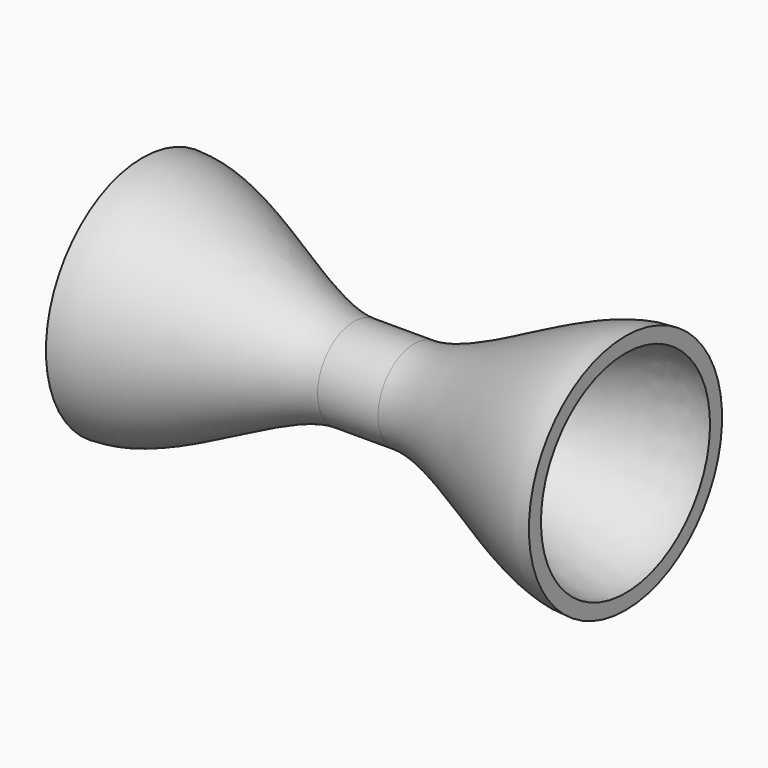
from build123d import *


# Not quite as in the source:
# - the dataset's text gives a spline's control points without its knots; the knots are read off the source's solid


with BuildPart() as f1:
    # F0 (on Front) → F1 (revolve)
    with BuildSketch(Plane.XZ):
        with BuildLine():
            Line((-66.7312243659, 73.4475515783), (-66.7312243659, 70.2725515783))
            add(Edge.make_bspline(
                [(-22.2812243659, 54.3975515783), (-34.9812243659, 54.3975515783), (-54.0312243659, 70.2725515783), (-66.7312243659, 70.2725515783)],
                knots=[0, 0, 0, 0, 47.1997682727, 47.1997682727, 47.1997682727, 47.1997682727], degree=3))
            Line((-22.2812243659, 54.3975515783), (-15.9312243659, 54.3975515783))
            Line((-15.9312243659, 54.3975515783), (-9.5812243659, 54.3975515783))
            add(Edge.make_bspline(
                [(-9.5812243659, 54.3975515783), (3.1187756341, 54.3975515783), (22.1687756341, 70.2725515783), (34.8687756341, 70.2725515783)],
                knots=[0, 0, 0, 0, 47.1997682727, 47.1997682727, 47.1997682727, 47.1997682727], degree=3))
            Line((34.8687756341, 70.2725515783), (34.8687756341, 73.4475515783))
            add(Edge.make_bspline(
                [(-9.5812243659, 57.5725515783), (-8.9528389492, 57.5725515783), (-7.604333407, 57.6714587753), (-4.5835276431, 58.2645427279), (-0.3121287775, 59.6981220412), (5.3075788443, 62.217263906), (11.2054567804, 65.1653736616), (17.2138288443, 68.170388906), (23.2027149725, 70.8602314162), (28.1090504819, 72.5272380404), (31.983947843, 73.2984119003), (33.9096610508, 73.4475515783), (34.8687756341, 73.4475515783)],
                knots=[0, 0, 0, 0, 0.0625, 0.125, 0.25, 0.375, 0.5, 0.625, 0.75, 0.875, 0.9375, 1, 1, 1, 1], degree=3))
            Line((-9.5812243659, 57.5725515783), (-15.9312243659, 57.5725515783))
            Line((-15.9312243659, 57.5725515783), (-22.2812243659, 57.5725515783))
            add(Edge.make_bspline(
                [(-22.2812243659, 57.5725515783), (-22.9096097826, 57.5725515783), (-24.2581153248, 57.6714587753), (-27.2789210887, 58.2645427279), (-31.5503199543, 59.6981220412), (-37.1700275761, 62.217263906), (-43.0679055123, 65.1653736616), (-49.0762775761, 68.170388906), (-55.0651637043, 70.8602314162), (-59.9714992137, 72.5272380404), (-63.8463965748, 73.2984119003), (-65.7721097826, 73.4475515783), (-66.7312243659, 73.4475515783)],
                knots=[0, 0, 0, 0, 0.0625, 0.125, 0.25, 0.375, 0.5, 0.625, 0.75, 0.875, 0.9375, 1, 1, 1, 1], degree=3))
        make_face()
    revolve(axis=Axis((-44.5062243659, 0, 48.0475515783), (1, 0, 0)))


solid = f1.part
